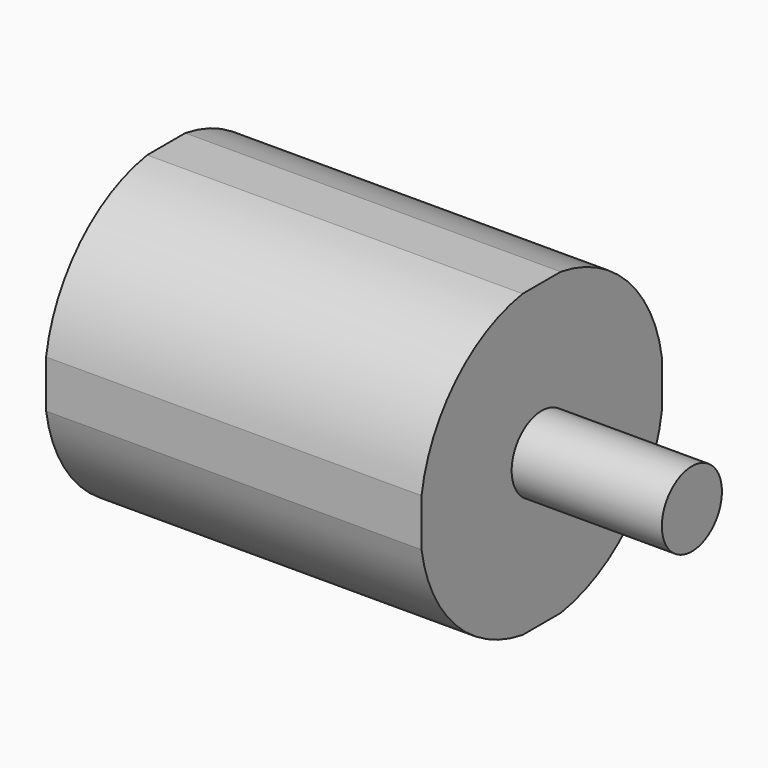
from build123d import *

# Parameters (mm, degrees)
F0_R     = 40.5
F1_DEPTH = 100
F2_W     = 90
F2_H     = 90
F3_DEPTH = 100.001
F4_R     = 10
F5_DEPTH = 40


with BuildPart() as f1:
    # F0 (on Right) → F1 (new body)
    with BuildSketch(Plane.YZ):
        Circle(F0_R)
    extrude(amount=F1_DEPTH)

    # F2 (on face) → F3 (cut, through all)
    with BuildSketch(Plane.YZ.offset(100)):
        Rectangle(F2_W, F2_H)
        with BuildLine():
            Line((40, -6.3442887702), (40, -40))
            Line((40, -40), (6.3442887702, -40))
            ThreePointArc((6.3442887702, -40), (0, -40.5), (-6.3442887702, -40))
            Line((-6.3442887702, -40), (-40, -40))
            Line((-40, -40), (-40, -6.3442887702))
            ThreePointArc((-40, -6.3442887702), (-40.5, 0), (-40, 6.3442887702))
            Line((-40, 6.3442887702), (-40, 40))
            Line((-40, 40), (-6.3442887702, 40))
            ThreePointArc((-6.3442887702, 40), (0, 40.5), (6.3442887702, 40))
            Line((6.3442887702, 40), (40, 40))
            Line((40, 40), (40, 6.3442887702))
            ThreePointArc((40, 6.3442887702), (40.3748065011, 3.1819805153), (40.5, 0))
            ThreePointArc((40.5, 0), (40.3748065011, -3.1819805153), (40, -6.3442887702))
        make_face(mode=Mode.SUBTRACT)
        with BuildLine():
            ThreePointArc((-6.3442887702, -40), (0, -40.5), (6.3442887702, -40))
            Line((6.3442887702, -40), (-6.3442887702, -40))
        make_face()
        with BuildLine():
            Line((40, 6.3442887702), (40, -6.3442887702))
            ThreePointArc((40, -6.3442887702), (40.3748065011, -3.1819805153), (40.5, 0))
            ThreePointArc((40.5, 0), (40.3748065011, 3.1819805153), (40, 6.3442887702))
        make_face()
        with BuildLine():
            ThreePointArc((-40, 6.3442887702), (-40.5, 0), (-40, -6.3442887702))
            Line((-40, -6.3442887702), (-40, 6.3442887702))
        make_face()
        with BuildLine():
            Line((-6.3442887702, 40), (6.3442887702, 40))
            ThreePointArc((6.3442887702, 40), (0, 40.5), (-6.3442887702, 40))
        make_face()
    extrude(amount=-F3_DEPTH, mode=Mode.SUBTRACT)

    # F4 (on face) → F5 (join)
    with BuildSketch(Plane.YZ.offset(100)):
        Circle(F4_R)
    extrude(amount=F5_DEPTH)


solid = f1.part
